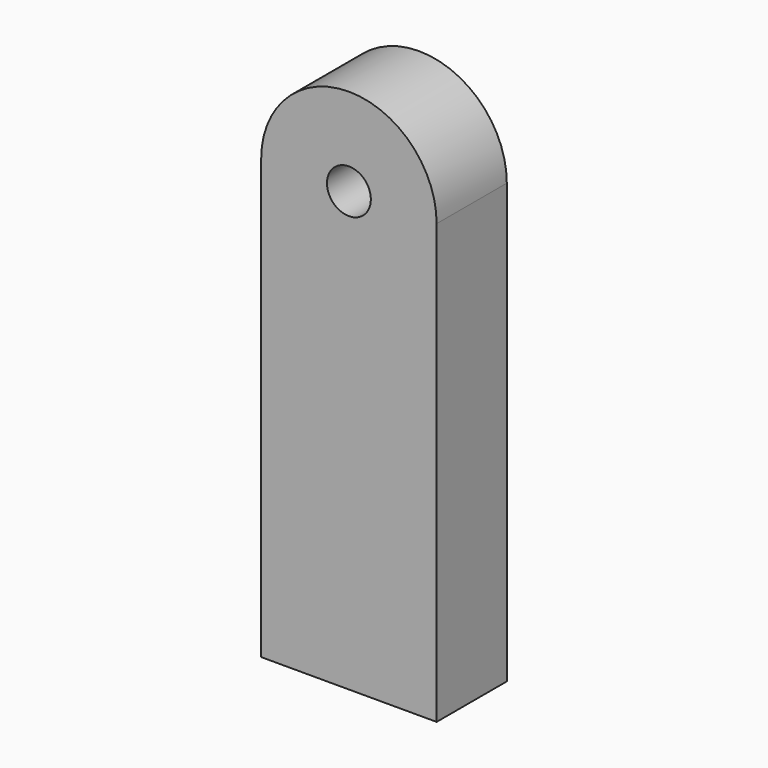
from build123d import *

# Parameters (mm, degrees)
F0_R     = 2.5
F1_DEPTH = 5


with BuildPart() as f1:
    # F0 (on Front) → F1 (new body, symmetric)
    with BuildSketch(Plane.XZ):
        with BuildLine():
            Line((-10, 25), (-10, -25))
            Line((-10, -25), (10, -25))
            Line((10, -25), (10, 25))
            ThreePointArc((10, 25), (0, 35), (-10, 25))
        make_face()
        with Locations((0, 25)):
            Circle(F0_R, mode=Mode.SUBTRACT)
    extrude(amount=F1_DEPTH, both=True)


solid = f1.part
